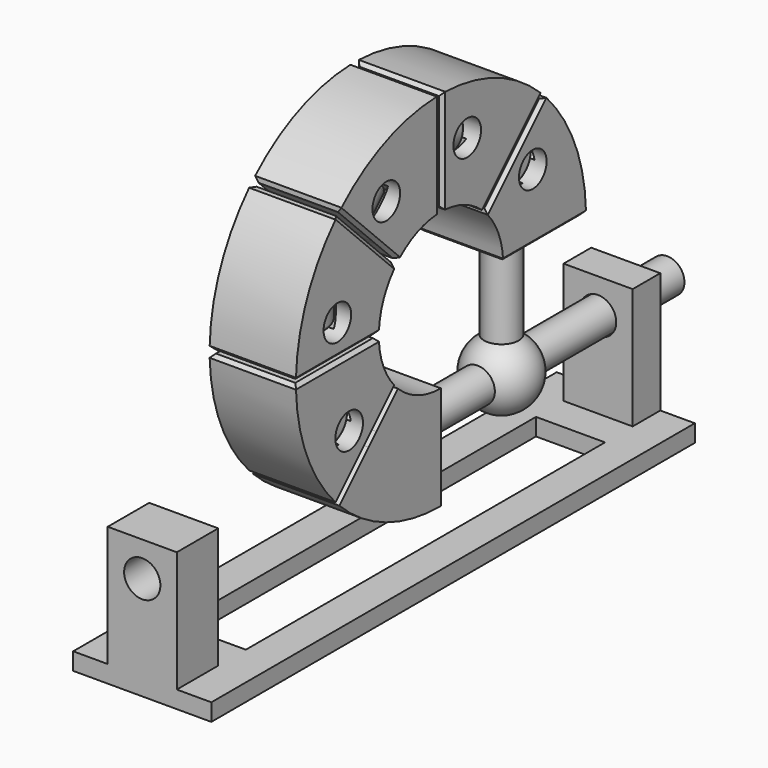
from build123d import *

# Parameters (mm, degrees)
F1_DEPTH     = 12.5
F0_W         = 37.5
F0_H         = 5
F0_W_2       = 2.5
F4_DEPTH     = 12.5
F6_D         = 10
F10_T1_DEPTH = 35.1465412112
F10_T3_DEPTH = 29.9359372009
F10_T5_DEPTH = 30.2892475518
F10_T7_DEPTH = 35.1465412112
F0_W_3       = 4
F0_H_2       = 0.5
F14_COUNT    = 5
F14_ANGLE    = 180
F0_W_4       = 5
F0_H_3       = 22.5
F0_W_5       = 10
F0_H_4       = 1.4819427681
F0_H_5       = 23.9819427681
F15_DEPTH    = 15
F0_H_6       = 4.5
F19_W        = 35
F19_H        = 5
F19_W_2      = 10
F19_W_3      = 15
F21_DEPTH    = 20
F23_D        = 10.5
F23_DEPTH    = 10
F23_TIP      = 3.1545182499
F25_D        = 10.5
F25_DEPTH    = 30
F25_TIP      = 3.1545182499
F26_W        = 20
F26_H        = 130
F27_DEPTH    = 5
F28_W        = 10
F28_H        = 35
F29_DEPTH    = 190.0010001


# Not quite as in the source:
# - a fillet or chamfer that OpenCascade refuses, or shapes differently, is made with other operations: its cross-section is extruded or revolved along the edge and cut away or added


with BuildPart() as f1:
    # F0 (on Right) → F1 (new body, symmetric)
    with BuildSketch(Plane.YZ):
        with BuildLine():
            Line((0, 20), (0, 30))
            ThreePointArc((0, 30), (-8.3788614978, 31.6183171176), (-15.55242033, 36.2404728888))
            Line((-15.55242033, 36.2404728888), (-23.3345237792, 28.4583694397))
            Line((-23.3345237792, 28.4583694397), (-26.1629509039, 25.6299423149))
            Line((-26.1629509039, 25.6299423149), (-28.9913780286, 22.8015151902))
            Line((-28.9913780286, 22.8015151902), (-36.7678689959, 15.0250242229))
            ThreePointArc((-36.7678689959, 15.0250242229), (-19.859679903, 3.9012025442), (0, 0))
            Line((0, 0), (0, 10))
            Line((0, 10), (0, 15))
            Line((0, 15), (0, 20))
        make_face()
    extrude(amount=F1_DEPTH, both=True)

    # F0 (on Right) → F2 (revolve)
    with BuildSketch(Plane.YZ):
        Polygon((-26.1629509039, 25.6299423149), (-23.3345237792, 28.4583694397), (-24.0416305603, 29.1654762208), (-26.8700576851, 26.3370490961), (-26.5165042945, 25.9834957055), align=None)
        with BuildLine():
            Line((-26.8700576851, 26.3370490961), (-24.0416305603, 29.1654762208))
            Line((-24.0416305603, 29.1654762208), (-27.9307178569, 33.0545635174))
            Line((-27.9307178569, 33.0545635174), (-25.1022907321, 35.8829906421))
            ThreePointArc((-25.1022907321, 35.8829906421), (-24.8093975133, 36.5900974233), (-25.1022907321, 37.2972042045))
            Line((-25.1022907321, 37.2972042045), (-28.6378246381, 40.8327381104))
            ThreePointArc((-28.6378246381, 40.8327381104), (-29.3449314192, 41.1256313292), (-30.0520382004, 40.8327381104))
            Line((-30.0520382004, 40.8327381104), (-35.7088924499, 35.1758838609))
            Line((-35.7088924499, 35.1758838609), (-26.8700576851, 26.3370490961))
        make_face()
    revolve(axis=Axis((0, -31.2894750675, 30.7564664785), (0, -0.7071067812, 0.7071067812)))

    # F0 (on Right) → F3 (revolve)
    with BuildSketch(Plane.YZ):
        with Locations((18.75, 17.5)):
            Rectangle(F0_W, F0_H)
        with Locations((38.75, 17.5)):
            Rectangle(F0_W_2, F0_H)
    revolve(axis=Axis((0, 20, 15), (0, 1, 0)))


with BuildPart() as f4:
    # F0 (on Right) → F4 (new body, symmetric)
    with BuildSketch(Plane.YZ):
        with BuildLine():
            Line((-22.9809703886, 30.2261363926), (-16.2595271112, 36.94757967))
            ThreePointArc((-16.2595271112, 36.94757967), (-20.7872894815, 43.8896227718), (-22.4944437584, 52))
            Line((-22.4944437584, 52), (-33.5, 52))
            Line((-33.5, 52), (-37.5, 52))
            Line((-37.5, 52), (-41.5, 52))
            Line((-41.5, 52), (-52.4976189936, 52))
            ThreePointArc((-52.4976189936, 52), (-48.5036754568, 32.4091198008), (-37.4749757771, 15.7321310041))
            Line((-37.4749757771, 15.7321310041), (-30.7591449816, 22.4479617996))
            ThreePointArc((-30.7591449816, 22.4479617996), (-30.4662517628, 23.1550685808), (-30.7591449816, 23.8621753619))
            Line((-30.7591449816, 23.8621753619), (-32.8804653252, 25.9834957055))
            ThreePointArc((-32.8804653252, 25.9834957055), (-33.5875721064, 26.2763889243), (-34.2946788875, 25.9834957055))
            Line((-34.2946788875, 25.9834957055), (-37.1231060123, 23.1550685808))
            Line((-37.1231060123, 23.1550685808), (-42.7799602618, 28.8119228303))
            Line((-42.7799602618, 28.8119228303), (-36.0624458405, 35.5294372515))
            Line((-36.0624458405, 35.5294372515), (-29.3449314192, 42.2469516728))
            Line((-29.3449314192, 42.2469516728), (-23.6880771697, 36.5900974233))
            Line((-23.6880771697, 36.5900974233), (-26.5165042945, 33.7616702986))
            ThreePointArc((-26.5165042945, 33.7616702986), (-26.8093975133, 33.0545635174), (-26.5165042945, 32.3474567362))
            Line((-26.5165042945, 32.3474567362), (-24.3951839509, 30.2261363926))
            ThreePointArc((-24.3951839509, 30.2261363926), (-23.6880771697, 29.9332431738), (-22.9809703886, 30.2261363926))
        make_face()
        with BuildLine():
            Line((-27.9307178569, 33.0545635174), (-24.0416305603, 29.1654762208))
            Line((-24.0416305603, 29.1654762208), (-22.9809703886, 30.2261363926))
            ThreePointArc((-22.9809703886, 30.2261363926), (-23.6880771697, 29.9332431738), (-24.3951839509, 30.2261363926))
            Line((-24.3951839509, 30.2261363926), (-26.5165042945, 32.3474567362))
            ThreePointArc((-26.5165042945, 32.3474567362), (-26.8093975133, 33.0545635174), (-26.5165042945, 33.7616702986))
            Line((-26.5165042945, 33.7616702986), (-23.6880771697, 36.5900974233))
            Line((-23.6880771697, 36.5900974233), (-29.3449314192, 42.2469516728))
            Line((-29.3449314192, 42.2469516728), (-36.0624458405, 35.5294372515))
            Line((-36.0624458405, 35.5294372515), (-35.7088924499, 35.1758838609))
            Line((-35.7088924499, 35.1758838609), (-30.0520382004, 40.8327381104))
            ThreePointArc((-30.0520382004, 40.8327381104), (-29.3449314192, 41.1256313292), (-28.6378246381, 40.8327381104))
            Line((-28.6378246381, 40.8327381104), (-25.1022907321, 37.2972042045))
            ThreePointArc((-25.1022907321, 37.2972042045), (-24.8093975133, 36.5900974233), (-25.1022907321, 35.8829906421))
            Line((-25.1022907321, 35.8829906421), (-27.9307178569, 33.0545635174))
        make_face()
        with BuildLine():
            Line((-26.8700576851, 26.3370490961), (-24.0416305603, 29.1654762208))
            Line((-24.0416305603, 29.1654762208), (-27.9307178569, 33.0545635174))
            Line((-27.9307178569, 33.0545635174), (-25.1022907321, 35.8829906421))
            ThreePointArc((-25.1022907321, 35.8829906421), (-24.8093975133, 36.5900974233), (-25.1022907321, 37.2972042045))
            Line((-25.1022907321, 37.2972042045), (-28.6378246381, 40.8327381104))
            ThreePointArc((-28.6378246381, 40.8327381104), (-29.3449314192, 41.1256313292), (-30.0520382004, 40.8327381104))
            Line((-30.0520382004, 40.8327381104), (-35.7088924499, 35.1758838609))
            Line((-35.7088924499, 35.1758838609), (-26.8700576851, 26.3370490961))
        make_face()
        with BuildLine():
            Line((-29.6984848098, 23.5086219714), (-26.8700576851, 26.3370490961))
            Line((-26.8700576851, 26.3370490961), (-35.7088924499, 35.1758838609))
            Line((-35.7088924499, 35.1758838609), (-41.3657466994, 29.5190296114))
            ThreePointArc((-41.3657466994, 29.5190296114), (-41.6586399182, 28.8119228303), (-41.3657466994, 28.1048160491))
            Line((-41.3657466994, 28.1048160491), (-37.8302127935, 24.5692821431))
            ThreePointArc((-37.8302127935, 24.5692821431), (-37.1231060123, 24.2763889243), (-36.4159992311, 24.5692821431))
            Line((-36.4159992311, 24.5692821431), (-33.5875721064, 27.3977092679))
            Line((-33.5875721064, 27.3977092679), (-29.6984848098, 23.5086219714))
        make_face()
        with BuildLine():
            Line((-41.3657466994, 29.5190296114), (-35.7088924499, 35.1758838609))
            Line((-35.7088924499, 35.1758838609), (-36.0624458405, 35.5294372515))
            Line((-36.0624458405, 35.5294372515), (-42.7799602618, 28.8119228303))
            Line((-42.7799602618, 28.8119228303), (-37.1231060123, 23.1550685808))
            Line((-37.1231060123, 23.1550685808), (-34.2946788875, 25.9834957055))
            ThreePointArc((-34.2946788875, 25.9834957055), (-33.5875721064, 26.2763889243), (-32.8804653252, 25.9834957055))
            Line((-32.8804653252, 25.9834957055), (-30.7591449816, 23.8621753619))
            ThreePointArc((-30.7591449816, 23.8621753619), (-30.4662517628, 23.1550685808), (-30.7591449816, 22.4479617996))
            Line((-30.7591449816, 22.4479617996), (-29.6984848098, 23.5086219714))
            Line((-29.6984848098, 23.5086219714), (-33.5875721064, 27.3977092679))
            Line((-33.5875721064, 27.3977092679), (-36.4159992311, 24.5692821431))
            ThreePointArc((-36.4159992311, 24.5692821431), (-37.1231060123, 24.2763889243), (-37.8302127935, 24.5692821431))
            Line((-37.8302127935, 24.5692821431), (-41.3657466994, 28.1048160491))
            ThreePointArc((-41.3657466994, 28.1048160491), (-41.6586399182, 28.8119228303), (-41.3657466994, 29.5190296114))
        make_face()
    extrude(amount=F4_DEPTH, both=True)

    # F6 (through all)
    with Locations(Plane.YZ.offset(12.5)):
        with Locations((-33.2340187158, 32.7010101268)):
            Hole(F6_D / 2)

    # F10: chamfer of 1 on 8 edges, made by hand

    # F10_s2 → F10_t1 (cut)
    with BuildSketch(Plane(origin=(0, -12.6898768664, -12.6898768664), x_dir=(1, 0, 0), z_dir=(0, 0.7071067812, 0.7071067812))):
        Polygon((-12.5, -38.6231060123), (-11.5, -37.6231060123), (-12.5, -37.6231060123), align=None)
        Polygon((12.5, -38.6231060123), (11.5, -37.6231060123), (12.5, -37.6231060123), align=None)
    extrude(amount=F10_T1_DEPTH, mode=Mode.SUBTRACT)

    # F10_s4 → F10_t3 (cut)
    with BuildSketch(Plane.YZ.offset(-14.9679686004)):
        with BuildLine():
            Line((-16.8929847992, 37.6380665936), (-16.9366773424, 36.2704294388))
            Line((-16.9366773424, 36.2704294388), (-16.2595271112, 36.94757967))
            ThreePointArc((-16.2595271112, 36.94757967), (-16.5895216397, 37.3000732974), (-16.8929847992, 37.6380665936))
        make_face()
        with BuildLine():
            Line((-22.4541179992, 51.0638297872), (-23.4520787991, 52))
            Line((-23.4520787991, 52), (-22.4944437584, 52))
            ThreePointArc((-22.4944437584, 52), (-22.4785344931, 51.5174079968), (-22.4541179992, 51.0638297872))
        make_face()
    extrude(amount=F10_T3_DEPTH, mode=Mode.SUBTRACT)

    # F10_s6 → F10_t5 (cut)
    with BuildSketch(Plane.YZ.offset(-15.1446237759)):
        with BuildLine():
            Line((-36.754102837, 16.4530039442), (-38.1886117467, 16.4738992832))
            ThreePointArc((-38.1886117467, 16.4738992832), (-37.8433662407, 16.1114079474), (-37.4749757771, 15.7321310041))
            Line((-37.4749757771, 15.7321310041), (-36.754102837, 16.4530039442))
        make_face()
        with BuildLine():
            Line((-51.4781507049, 52), (-52.4777264468, 50.9708737864))
            ThreePointArc((-52.4777264468, 50.9708737864), (-52.48992109, 51.4713193065), (-52.4976189936, 52))
            Line((-52.4976189936, 52), (-51.4781507049, 52))
        make_face()
    extrude(amount=F10_T5_DEPTH, mode=Mode.SUBTRACT)

    # F10_s8 → F10_t7 (cut)
    with BuildSketch(Plane.XZ.offset(19.9227607704)):
        Polygon((-12.5, 51), (-11.5, 52), (-12.5, 52), align=None)
        Polygon((11.5, 52), (12.5, 51), (12.5, 52), align=None)
    extrude(amount=F10_T7_DEPTH, mode=Mode.SUBTRACT)

    # F0 (on Right) → F11 (revolve)
    with BuildSketch(Plane.YZ):
        with BuildLine():
            Line((-37.5, 52.5), (-33.5, 52.5))
            Line((-33.5, 52.5), (-33.5, 58.5))
            Line((-33.5, 58.5), (-29.5, 58.5))
            ThreePointArc((-29.5, 58.5), (-28.7928932188, 58.7928932188), (-28.5, 59.5))
            Line((-28.5, 59.5), (-28.5, 64.5))
            ThreePointArc((-28.5, 64.5), (-28.7928932188, 65.2071067812), (-29.5, 65.5))
            Line((-29.5, 65.5), (-37.5, 65.5))
            Line((-37.5, 65.5), (-37.5, 52.5))
        make_face()
        with Locations((-35.5, 52.25)):
            Rectangle(F0_W_3, F0_H_2)
    revolve(axis=Axis((0, -37.5, 58.75), (0, 0, 1)))

    # F0 (on Right) → F12 (revolve, cut)
    with BuildSketch(Plane.YZ):
        with BuildLine():
            Line((-26.8700576851, 26.3370490961), (-24.0416305603, 29.1654762208))
            Line((-24.0416305603, 29.1654762208), (-27.9307178569, 33.0545635174))
            Line((-27.9307178569, 33.0545635174), (-25.1022907321, 35.8829906421))
            ThreePointArc((-25.1022907321, 35.8829906421), (-24.8093975133, 36.5900974233), (-25.1022907321, 37.2972042045))
            Line((-25.1022907321, 37.2972042045), (-28.6378246381, 40.8327381104))
            ThreePointArc((-28.6378246381, 40.8327381104), (-29.3449314192, 41.1256313292), (-30.0520382004, 40.8327381104))
            Line((-30.0520382004, 40.8327381104), (-35.7088924499, 35.1758838609))
            Line((-35.7088924499, 35.1758838609), (-26.8700576851, 26.3370490961))
        make_face()
        with BuildLine():
            Line((-27.9307178569, 33.0545635174), (-24.0416305603, 29.1654762208))
            Line((-24.0416305603, 29.1654762208), (-22.9809703886, 30.2261363926))
            ThreePointArc((-22.9809703886, 30.2261363926), (-23.6880771697, 29.9332431738), (-24.3951839509, 30.2261363926))
            Line((-24.3951839509, 30.2261363926), (-26.5165042945, 32.3474567362))
            ThreePointArc((-26.5165042945, 32.3474567362), (-26.8093975133, 33.0545635174), (-26.5165042945, 33.7616702986))
            Line((-26.5165042945, 33.7616702986), (-23.6880771697, 36.5900974233))
            Line((-23.6880771697, 36.5900974233), (-29.3449314192, 42.2469516728))
            Line((-29.3449314192, 42.2469516728), (-36.0624458405, 35.5294372515))
            Line((-36.0624458405, 35.5294372515), (-35.7088924499, 35.1758838609))
            Line((-35.7088924499, 35.1758838609), (-30.0520382004, 40.8327381104))
            ThreePointArc((-30.0520382004, 40.8327381104), (-29.3449314192, 41.1256313292), (-28.6378246381, 40.8327381104))
            Line((-28.6378246381, 40.8327381104), (-25.1022907321, 37.2972042045))
            ThreePointArc((-25.1022907321, 37.2972042045), (-24.8093975133, 36.5900974233), (-25.1022907321, 35.8829906421))
            Line((-25.1022907321, 35.8829906421), (-27.9307178569, 33.0545635174))
        make_face()
    revolve(axis=Axis((0, -31.2894750675, 30.7564664785), (0, -0.7071067812, 0.7071067812)), mode=Mode.SUBTRACT)


with BuildPart() as f14_1:
    # F14: instance of F4
    add(f4.part.rotate(Axis((0, 0, 52.5), (-1, 0, 0)), 1 * F14_ANGLE / (F14_COUNT - 1)))


with BuildPart() as f14_2:
    # F14: instance of F4
    add(f4.part.rotate(Axis((0, 0, 52.5), (-1, 0, 0)), 2 * F14_ANGLE / (F14_COUNT - 1)))


with BuildPart() as f14_3:
    # F14: instance of F4
    add(f4.part.rotate(Axis((0, 0, 52.5), (-1, 0, 0)), 3 * F14_ANGLE / (F14_COUNT - 1)))


with BuildPart() as f14_4:
    # F14: instance of F4
    add(f4.part.rotate(Axis((0, 0, 52.5), (-1, 0, 0)), 4 * F14_ANGLE / (F14_COUNT - 1)))

    # F0 (on Right) → F15 (cut, symmetric)
    with BuildSketch(Plane.YZ):
        Polygon((37.5, 52.5), (37.5, 30), (40, 30), (40, 28.5180572319), (42.5, 28.5180572319), (42.5, 52.5), align=None)
        with Locations((35, 41.25)):
            Rectangle(F0_W_4, F0_H_3)
        with Locations((27.5, 41.25)):
            Rectangle(F0_W_5, F0_H_3)
        with Locations((27.5, 29.2590286159)):
            Rectangle(F0_W_5, F0_H_4)
        with Locations((35, 29.2590286159)):
            Rectangle(F0_W_4, F0_H_4)
        with Locations((38.75, 29.2590286159)):
            Rectangle(F0_W_2, F0_H_4)
        with Locations((47.5, 40.5090286159)):
            Rectangle(F0_W_5, F0_H_5)
        with BuildLine():
            ThreePointArc((22.4944437584, 53), (22.4986108967, 52.7500154354), (22.5, 52.5))
            Line((22.5, 52.5), (32.5, 52.5))
            Line((32.5, 52.5), (32.5, 53))
            Line((32.5, 53), (22.4944437584, 53))
        make_face()
        with Locations((35, 52.75)):
            Rectangle(F0_W_4, F0_H_2)
        with Locations((40, 52.75)):
            Rectangle(F0_W_4, F0_H_2)
        with BuildLine():
            Line((42.5, 53), (42.5, 52.5))
            Line((42.5, 52.5), (52.5, 52.5))
            ThreePointArc((52.5, 52.5), (52.499404745, 52.7500028346), (52.4976189936, 53))
            Line((52.4976189936, 53), (42.5, 53))
        make_face()
    extrude(amount=F15_DEPTH, both=True, mode=Mode.SUBTRACT)

    # F0 (on Right) → F18 (revolve)
    with BuildSketch(Plane.YZ):
        Polygon((37.5, 52.5), (37.5, 30), (40, 30), (40, 28.5180572319), (42.5, 28.5180572319), (42.5, 52.5), align=None)
        with Locations((38.75, 29.2590286159)):
            Rectangle(F0_W_2, F0_H_4)
        with BuildLine():
            Line((37.5, 28.5180572319), (37.5, 25))
            ThreePointArc((37.5, 25), (38.7600429248, 24.9202969627), (40, 24.6824583655))
            Line((40, 24.6824583655), (40, 28.5180572319))
            Line((40, 28.5180572319), (37.5, 28.5180572319))
        make_face()
        with BuildLine():
            Line((40, 28.5180572319), (40, 24.6824583655))
            ThreePointArc((40, 24.6824583655), (40.3127293707, 24.596278106), (40.6224989992, 24.5))
            Line((40.6224989992, 24.5), (42.5, 24.5))
            Line((42.5, 24.5), (42.5, 25))
            Line((42.5, 25), (42.5, 28.5180572319))
            Line((42.5, 28.5180572319), (40, 28.5180572319))
        make_face()
        with Locations((40, 52.75)):
            Rectangle(F0_W_4, F0_H_2)
    revolve(axis=Axis((0, 37.5, 34), (0, 0, -1)))


with BuildPart() as f16:
    # F0 (on Right) → F16 (revolve)
    with BuildSketch(Plane.YZ):
        with Locations((38.75, 12.5)):
            Rectangle(F0_W_2, F0_H)
        with BuildLine():
            Line((40, 24.5), (40, 20))
            Line((40, 20), (40, 15))
            Line((40, 15), (40, 10))
            Line((40, 10), (37.5, 10))
            Line((37.5, 10), (37.5, 5))
            ThreePointArc((37.5, 5), (47.3742088291, 13.4188611699), (40.6224989992, 24.5))
            Line((40.6224989992, 24.5), (40, 24.5))
        make_face()
        with BuildLine():
            Line((37.5, 25), (37.5, 24.5))
            Line((37.5, 24.5), (40, 24.5))
            Line((40, 24.5), (40, 24.6824583655))
            ThreePointArc((40, 24.6824583655), (38.7600429248, 24.9202969627), (37.5, 25))
        make_face()
        with Locations((38.75, 22.25)):
            Rectangle(F0_W_2, F0_H_6)
        with Locations((38.75, 17.5)):
            Rectangle(F0_W_2, F0_H)
        with BuildLine():
            Line((40, 24.6824583655), (40, 24.5))
            Line((40, 24.5), (40.6224989992, 24.5))
            ThreePointArc((40.6224989992, 24.5), (40.3127293707, 24.596278106), (40, 24.6824583655))
        make_face()
    revolve(axis=Axis((0, 37.5, 34), (0, 0, -1)))

    # F19 (on Right) → F20 (revolve)
    with BuildSketch(Plane.YZ):
        with Locations((55, 17.5)):
            Rectangle(F19_W, F19_H)
        with Locations((77.5, 17.5)):
            Rectangle(F19_W_2, F19_H)
        with Locations((90, 17.5)):
            Rectangle(F19_W_3, F19_H)
    revolve(axis=Axis((0, 67.5, 15), (0, 1, 0)))


with BuildPart() as f17:
    # F0 (on Right) → F17 (revolve)
    with BuildSketch(Plane.YZ):
        with Locations((38.75, 22.25)):
            Rectangle(F0_W_2, F0_H_6)
    revolve(axis=Axis((0, 38.75, 15), (0, 1, 0)))


with BuildPart() as f21:
    # F19 (on Right) → F21 (new body, symmetric)
    with BuildSketch(Plane.YZ):
        Polygon((-92.5, -15), (82.5, -15), (82.5, 15), (72.5, 15), (72.5, -10), (-77.5, -10), (-77.5, 25), (-92.5, 25), align=None)
        with Locations((77.5, 17.5)):
            Rectangle(F19_W_2, F19_H)
        with Locations((77.5, 22.5)):
            Rectangle(F19_W_2, F19_H)
    extrude(amount=F21_DEPTH, both=True)

    # F23
    with Locations(Plane(origin=(0, 82.5, 0), x_dir=(-1, 0, 0), z_dir=(0, 1, 0))):
        with Locations((0, 15)):
            Hole(F23_D / 2, depth=F23_DEPTH)
            with Locations((0, 0, -(F23_DEPTH + F23_TIP / 2))):  # 118° drill point
                Cone(0, F23_D / 2, F23_TIP, mode=Mode.SUBTRACT)

    # F25
    with Locations(Plane.XZ.offset(92.5)):
        with Locations((0, 15)):
            Hole(F25_D / 2, depth=F25_DEPTH)
            with Locations((0, 0, -(F25_DEPTH + F25_TIP / 2))):  # 118° drill point
                Cone(0, F25_D / 2, F25_TIP, mode=Mode.SUBTRACT)

    # F26 (on face) → F27 (cut, through all)
    with BuildSketch(Plane.XY.offset(-10)):
        with Locations((0, -2.5)):
            Rectangle(F26_W, F26_H)
    extrude(amount=-F27_DEPTH, mode=Mode.SUBTRACT)

    # F28 (on face) → F29 (cut, through all)
    with BuildSketch(Plane.XZ.offset(92.5)):
        with Locations((-15, 7.5)):
            Rectangle(F28_W, F28_H)
        with Locations((15, 7.5)):
            Rectangle(F28_W, F28_H)
    extrude(amount=-F29_DEPTH, mode=Mode.SUBTRACT)


solid = Compound([f1.part, f4.part, f14_1.part, f14_2.part, f14_3.part, f14_4.part, f16.part, f17.part, f21.part])
